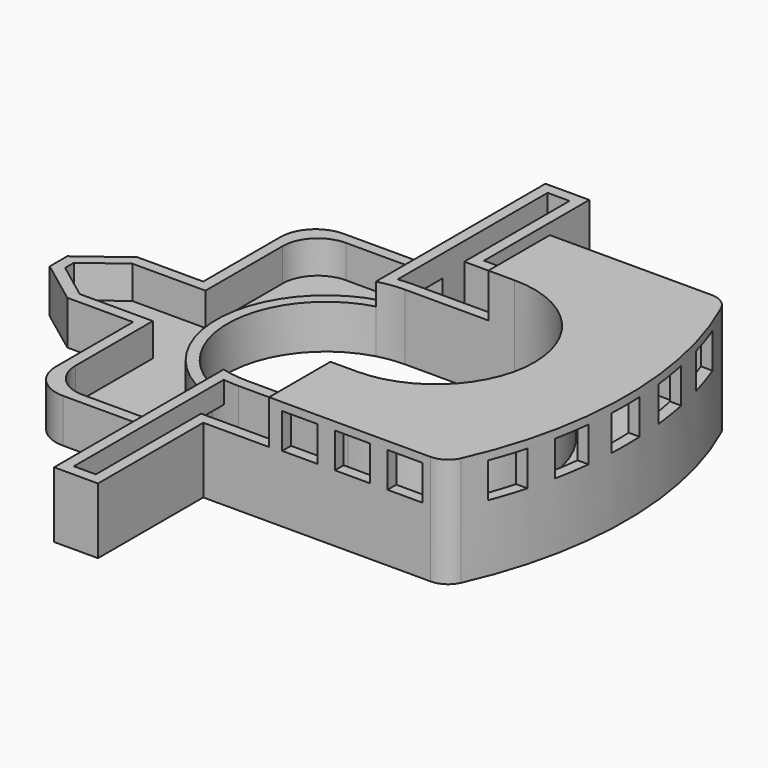
from build123d import *

# Parameters (mm, degrees)
F1_DEPTH    = 15.875
F2_DEPTH    = 9.525
F3_DEPTH    = 6.35
F4_T        = 1.5875
F4_T3_DEPTH = 12.7
F4_T5_DEPTH = 9.525
F5_W        = 5.08
F5_H        = 5.08
F6_DEPTH    = 1.778
F7_W        = 5.08
F7_H        = 5.08
F8_DEPTH    = 1.778
F10_W       = 5.08
F10_H       = 5.08
F11_DEPTH   = 7.62
F12_DEPTH   = 7.62
F13_R       = 5.08


# Not quite as in the source:
# - after a boolean that leaves OpenCascade's solid faulty, fix() repairs it
# - a shell that OpenCascade refuses in one call is made with other operations: the cavity is built on its own and cut out


with BuildPart() as f1:
    # F0 (on Top) → F1 (new body)
    with BuildSketch(Plane.XY):
        with BuildLine():
            Line((34.925, 50.8), (34.925, 39.6875))
            Line((34.925, 39.6875), (38.735, 39.6875))
            ThreePointArc((38.735, 39.6875), (53.0225, 25.4), (38.735, 11.1125))
            Line((38.735, 11.1125), (34.925, 11.1125))
            Line((34.925, 11.1125), (34.925, 0))
            Line((34.925, 0), (58.3165517951, 0))
            ThreePointArc((58.3165517951, 0), (60.0384373041, 0.5074664399), (61.2098981773, 1.8676470588))
            ThreePointArc((61.2098981773, 1.8676470588), (66.2796632983, 25.4), (61.2098981773, 48.9323529412))
            ThreePointArc((61.2098981773, 48.9323529412), (60.0384373041, 50.2925335601), (58.3165517951, 50.8))
            Line((58.3165517951, 50.8), (34.925, 50.8))
        make_face()
    extrude(amount=F1_DEPTH)

    # F0 (on Top) → F2 (join)
    with BuildSketch(Plane.XY):
        with BuildLine():
            Line((19.05, 69.85), (19.05, 50.8))
            Line((19.05, 50.8), (19.05, 39.1701327608))
            ThreePointArc((19.05, 39.1701327608), (20.9375166542, 39.557567377), (22.86, 39.6875))
            Line((22.86, 39.6875), (34.925, 39.6875))
            Line((34.925, 39.6875), (34.925, 50.8))
            Line((34.925, 50.8), (25.4, 50.8))
            Line((25.4, 50.8), (25.4, 69.85))
            Line((25.4, 69.85), (19.05, 69.85))
        make_face()
        with BuildLine():
            ThreePointArc((22.86, 11.1125), (20.9375166542, 11.242432623), (19.05, 11.6298672392))
            Line((19.05, 11.6298672392), (19.05, 0))
            Line((19.05, 0), (19.05, -19.05))
            Line((19.05, -19.05), (25.4, -19.05))
            Line((25.4, -19.05), (25.4, 0))
            Line((25.4, 0), (34.925, 0))
            Line((34.925, 0), (34.925, 11.1125))
            Line((34.925, 11.1125), (22.86, 11.1125))
        make_face()
    extrude(amount=F2_DEPTH)

    # F0 (on Top) → F3 (join)
    with BuildSketch(Plane.XY):
        with BuildLine():
            Line((19.05, 50.8), (0, 50.8))
            Line((0, 50.8), (0, 31.75))
            Line((0, 31.75), (0, 19.05))
            Line((0, 19.05), (0, 0))
            Line((0, 0), (19.05, 0))
            Line((19.05, 0), (19.05, 11.6298672392))
            ThreePointArc((19.05, 11.6298672392), (8.5725, 25.4), (19.05, 39.1701327608))
            Line((19.05, 39.1701327608), (19.05, 50.8))
        make_face()
        Polygon((0, 19.05), (0, 31.75), (-9.525, 31.75), (-15.875, 26.9875), (-15.875, 23.8125), (-9.525, 19.05), align=None)
    extrude(amount=F3_DEPTH)

    add(f1.part.fix(), mode=Mode.REPLACE)

    # F4: shell of thickness 1.5875, made by hand


with BuildPart() as f4_core1:
    # F4_t2: copy of F1
    add(f1.part)

    # the walls: a layer under each face that stays
    f4_faces = [f4_core1.faces().sort_by_distance(p)[0] for p in [
        (60.0384373041, 50.2925335601, 7.9375),
        (66.2796632983, 25.4, 7.9375),
        (41.8582758976, 50.8, 7.9375),
        (-2.1825561169, 25.4, 0),
        (40.1507772164, 8.4666666667, 15.875),
        (60.0384373041, 0.5074664399, 7.9375),
        (25.4, 60.325, 4.7625),
        (22.225, 69.85, 4.7625),
        (19.05, 54.5100663804, 4.7625),
        (20.9375166542, 39.557567377, 4.7625),
        (30.7975, 39.6875, 7.9375),
        (53.0225, 25.4, 7.9375),
        (30.7975, 11.1125, 7.9375),
        (20.9375166542, 11.242432623, 4.7625),
        (19.05, -3.7100663804, 4.7625),
        (22.225, -19.05, 4.7625),
        (25.4, -9.525, 4.7625),
        (41.8582758976, 0, 7.9375),
        (9.525, 50.8, 3.175),
        (0, 41.275, 3.175),
        (-4.7625, 31.75, 3.175),
        (-12.7, 29.36875, 3.175),
        (-15.875, 25.4, 3.175),
        (-12.7, 21.43125, 3.175),
        (-4.7625, 19.05, 3.175),
        (0, 9.525, 3.175),
        (9.525, 0, 3.175),
        (8.5725, 25.4, 3.175),
    ]]
    thicken(f4_faces, amount=-F4_T, mode=Mode.SUBTRACT)

    # F4_s4 → F4_t3 (cut)
    with BuildSketch(Plane.XY.offset(-1.5875)):
        Polygon((25.415875, 50.815875), (25.4, 49.2125), (23.8125, 49.2125), (23.8125, 50.8), align=None)
        Polygon((25.415875, -0.015875), (23.8125, 0), (23.8125, 1.5875), (25.4, 1.5875), align=None)
    extrude(amount=F4_T3_DEPTH, mode=Mode.SUBTRACT)

    # F4_s6 → F4_t5 (cut)
    with BuildSketch(Plane.XY.offset(-1.5875)):
        Polygon((19.034125, 50.815875), (20.6375, 50.8), (20.6375, 49.2125), (19.05, 49.2125), align=None)
        Polygon((19.034125, -0.015875), (20.6375, 0), (20.6375, 1.5875), (19.05, 1.5875), align=None)
        Polygon((-0.015875, 31.765875), (1.5875, 31.75), (1.5875, 30.1625), (0, 30.1625), align=None)
        Polygon((-0.015875, 19.034125), (0, 20.6375), (1.5875, 20.6375), (1.5875, 19.05), align=None)
    extrude(amount=F4_T5_DEPTH, mode=Mode.SUBTRACT)


with BuildPart() as f1_1:
    add(f1.part)

    # what is left inside the walls is the cavity
    f4_cavity = [f4_core1.part.solids().sort_by_distance(p)[0] for p in [
        (5.457416, 39.6875, 1.603375),
    ]]
    add(f4_cavity, mode=Mode.SUBTRACT)

    # F5 (on face) → F6 (cut)
    with BuildSketch(Plane(origin=(0, 50.8, 0), x_dir=(-1, 0, 0), z_dir=(0, 1, 0))):
        with Locations((-54.61, 12.192)):
            Rectangle(F5_W, F5_H)
        with Locations((-46.99, 12.192)):
            Rectangle(F5_W, F5_H)
        with Locations((-39.37, 12.192)):
            Rectangle(F5_W, F5_H)
    extrude(amount=-F6_DEPTH, mode=Mode.SUBTRACT)

    # F7 (on face) → F8 (cut)
    with BuildSketch(Plane.XZ):
        with Locations((39.37, 12.192)):
            Rectangle(F7_W, F7_H)
        with Locations((46.99, 12.192)):
            Rectangle(F7_W, F7_H)
        with Locations((54.61, 12.192)):
            Rectangle(F7_W, F7_H)
    extrude(amount=-F8_DEPTH, mode=Mode.SUBTRACT)

    # F10 (on offset) → F11 (cut)
    with BuildSketch(Plane.YZ.offset(66.294)):
        with Locations((7.62, 12.192)):
            Rectangle(F10_W, F10_H)
    extrude(amount=-F11_DEPTH, mode=Mode.SUBTRACT)

    # F10 (on offset) → F12 (cut)
    with BuildSketch(Plane.YZ.offset(66.294)):
        with Locations((16.51, 12.192)):
            Rectangle(F10_W, F10_H)
        with Locations((25.4, 12.192)):
            Rectangle(F10_W, F10_H)
        with Locations((34.29, 12.192)):
            Rectangle(F10_W, F10_H)
        with Locations((43.18, 12.192)):
            Rectangle(F10_W, F10_H)
    extrude(amount=-F12_DEPTH, mode=Mode.SUBTRACT)

    # F13
    f13_edges = [f1_1.edges().sort_by_distance(p)[0] for p in [
        (0, 0, 3.175),
        (1.5875, 1.5875, 3.96875),
        (0, 50.8, 3.175),
        (1.5875, 49.2125, 3.96875),
    ]]
    fillet(f13_edges, radius=F13_R)


solid = f1_1.part
